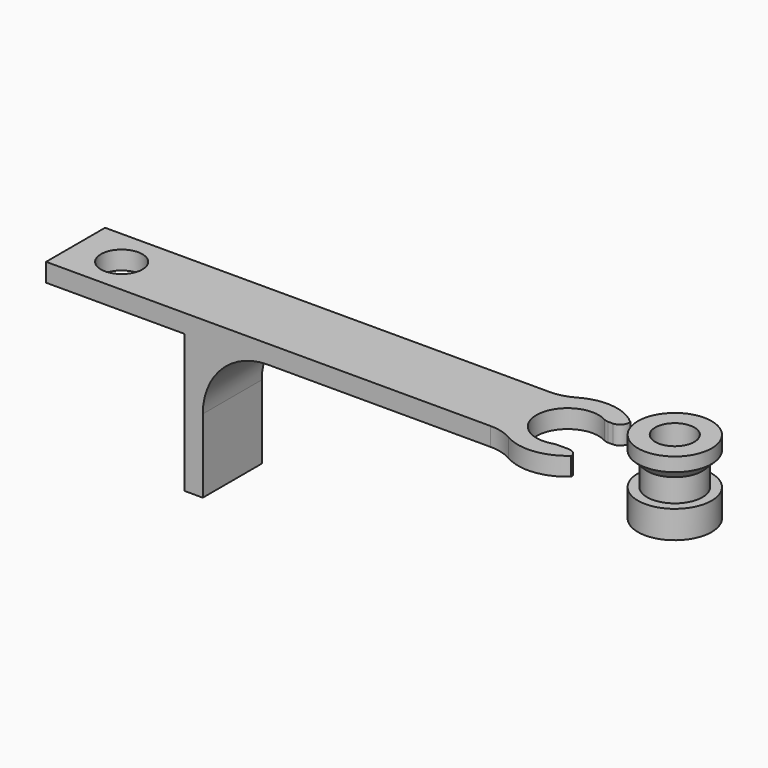
from build123d import *

# Parameters (mm, degrees)
F1_DEPTH       = 4
F2_R           = 5.375
F3_DEPTH       = 2
F5_DEPTH       = 17.001
F6_R           = 7
F7_T1_DEPTH    = 3.3790215822
F7_T3_DEPTH    = 2.8251909372
F7_T5_DEPTH    = 10.474284143
F7_T7_DEPTH    = 11.6759161977
F8_R           = 2.25
F9_DEPTH       = 17.001
F10_R          = 3
F10_R_2        = 2.125
F11_DEPTH      = 5
F11_DEPTH_BACK = 3
F10_R_3        = 4
F12_DEPTH      = 3
F13_R          = 4
F13_R_2        = 3
F14_DEPTH      = 2.5
F15_R          = 2.125
F15_R_2        = 1.5
F16_DEPTH      = 1
F17_SIZE       = 0.99999
F18_R          = 5


# Not quite as in the source:
# - a fillet or chamfer that OpenCascade refuses, or shapes differently, is made with other operations: its cross-section is extruded or revolved along the edge and cut away or added
# - a fillet or chamfer is up to 0.001 mm smaller than in the source, because OpenCascade refuses the exact size


with BuildPart() as f1:
    # F0 (on Front) → F1 (new body, symmetric)
    with BuildSketch(Plane.XZ):
        Polygon((0, -15), (0, 0), (40, 0), (40, 2), (0, 2), (-17, 2), (-17, 0), (-2, 0), (-2, -15), align=None)
    extrude(amount=F1_DEPTH, both=True)

    # F2 (on face) → F3 (join, through all)
    with BuildSketch(Plane.XY.offset(2)):
        with Locations((36.375, 0)):
            Circle(F2_R)
    extrude(amount=-F3_DEPTH)

    # F4 (on face) → F5 (cut, through all)
    with BuildSketch(Plane.XY.offset(2)):
        with BuildLine():
            Line((40.9448929828, 2.8296118331), (38.214543931, 2.8296118331))
            ThreePointArc((38.214543931, 2.8296118331), (33.0216111212, 0.3813240457), (37.5322656873, -3.1703881669))
            Line((37.5322656873, -3.1703881669), (40.7154220844, -3.1703881669))
            ThreePointArc((40.7154220844, -3.1703881669), (41.7460733238, -0.2054175034), (40.9448929828, 2.8296118331))
        make_face()
    extrude(amount=-F5_DEPTH, mode=Mode.SUBTRACT)

    # F6
    f6_edges = [f1.edges().sort_by_distance(p)[0] for p in [
        (0, 0, 0),
    ]]
    fillet(f6_edges, radius=F6_R)

    # F7: fillet of radius 1 on 4 edges, made by hand

    # F7_s2 → F7_t1 (cut)
    with BuildSketch(Plane.XY.offset(-0.6895107911)):
        with BuildLine():
            ThreePointArc((38.0068400766, 2.9542719855), (38.2406883263, 2.8612782522), (38.4903482474, 2.8296118331))
            Line((38.4903482474, 2.8296118331), (38.214543931, 2.8296118331))
            ThreePointArc((38.214543931, 2.8296118331), (38.1118108044, 2.8938060111), (38.0068400766, 2.9542719855))
        make_face()
    extrude(amount=F7_T1_DEPTH, mode=Mode.SUBTRACT)

    # F7_s4 → F7_t3 (cut)
    with BuildSketch(Plane.XY.offset(-0.4125954686)):
        with BuildLine():
            ThreePointArc((37.6973038748, -3.1703881669), (37.544384911, -3.1821494354), (37.3950629891, -3.2171565859))
            ThreePointArc((37.3950629891, -3.2171565859), (37.4639154525, -3.1945090605), (37.5322656873, -3.1703881669))
            Line((37.5322656873, -3.1703881669), (37.6973038748, -3.1703881669))
        make_face()
    extrude(amount=F7_T3_DEPTH, mode=Mode.SUBTRACT)

    # F7_s6 → F7_t5 (cut)
    with BuildSketch(Plane.XY.offset(-4.2371420715)):
        with BuildLine():
            ThreePointArc((40, -3.9686269666), (39.6523242288, -3.3952232811), (39.0205652559, -3.1703881669))
            Line((39.0205652559, -3.1703881669), (40.7154220844, -3.1703881669))
            ThreePointArc((40.7154220844, -3.1703881669), (40.3776595585, -3.5873864385), (40, -3.9686269666))
        make_face()
    extrude(amount=F7_T5_DEPTH, mode=Mode.SUBTRACT)

    # F7_s8 → F7_t7 (cut)
    with BuildSketch(Plane.XY.offset(-4.8379580989)):
        with BuildLine():
            ThreePointArc((40, 3.9686269666), (39.7643669944, 3.1734926113), (39.0097097432, 2.8296118331))
            Line((39.0097097432, 2.8296118331), (40.9448929828, 2.8296118331))
            ThreePointArc((40.9448929828, 2.8296118331), (40.5118353386, 3.4317952127), (40, 3.9686269666))
        make_face()
    extrude(amount=F7_T7_DEPTH, mode=Mode.SUBTRACT)

    # F8 (on face) → F9 (cut, through all)
    with BuildSketch(Plane.XY.offset(2)):
        with Locations((-12, 0)):
            Circle(F8_R)
    extrude(amount=-F9_DEPTH, mode=Mode.SUBTRACT)

    # F18
    f18_edges = [f1.edges().sort_by_distance(p)[0] for p in [
        (32.784648, 4, 1),
        (32.784648, -4, 1),
    ]]
    fillet(f18_edges, radius=F18_R)


with BuildPart() as f11:
    # F10 (on Top) → F11 (new body, two sides)
    with BuildSketch(Plane.XY) as f11_sk:
        with Locations((48, 0)):
            Circle(F10_R)
        with Locations((48, 0)):
            Circle(F10_R_2, mode=Mode.SUBTRACT)
    extrude(amount=F11_DEPTH)
    extrude(f11_sk.sketch, amount=-F11_DEPTH_BACK)

    # F10 (on Top) → F12 (join, through all)
    with BuildSketch(Plane.XY):
        with Locations((48, 0)):
            Circle(F10_R_3)
        with Locations((48, 0)):
            Circle(F10_R, mode=Mode.SUBTRACT)
    extrude(amount=-F12_DEPTH)

    # F13 (on face) → F14 (join)
    with BuildSketch(Plane.XY.offset(5)):
        with Locations((48, 0)):
            Circle(F13_R)
        with Locations((48, 0)):
            Circle(F13_R_2, mode=Mode.SUBTRACT)
    extrude(amount=-F14_DEPTH)

    # F15 (on face) → F16 (join)
    with BuildSketch(Plane(origin=(0, 0, -3), x_dir=(1, 0, 0), z_dir=(0, 0, -1))):
        with Locations((48, 0)):
            Circle(F15_R)
        with Locations((48, 0)):
            Circle(F15_R_2, mode=Mode.SUBTRACT)
    extrude(amount=-F16_DEPTH)

    # F17 (size 1 in the source; OpenCascade refuses exactly that, so slightly less here)
    f17_edges = [f11.edges().sort_by_distance(p)[0] for p in [
        (44, 0, 2.5),
    ]]
    chamfer(f17_edges, length=F17_SIZE)


solid = Compound([f1.part, f11.part])
